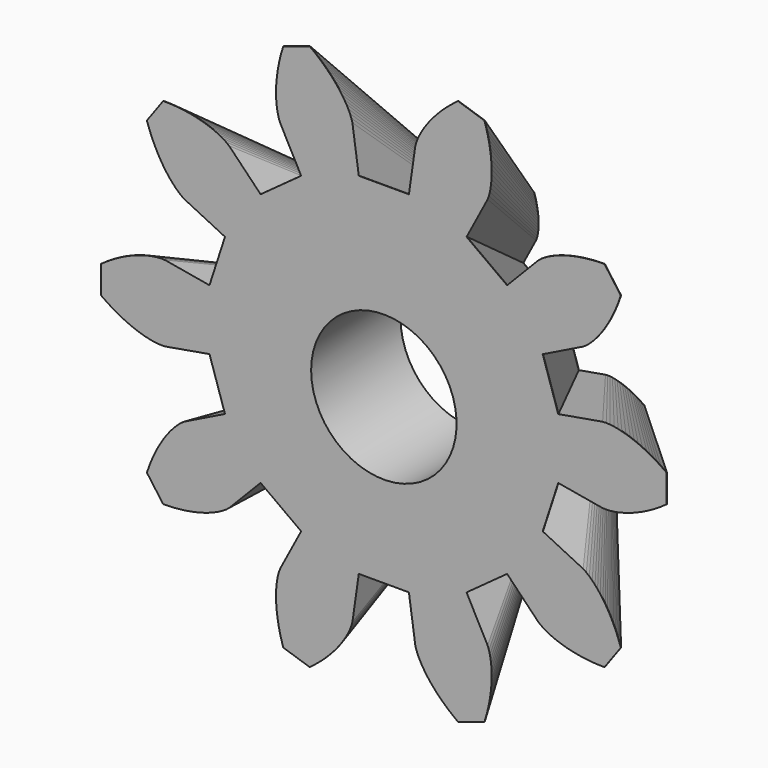
from build123d import *

# Parameters (mm, degrees)
F1_DEPTH = 0.01
F3_SCALE = 0.6058
F5_R     = 1.9570867443
F6_DEPTH = 3.011


# Not quite as in the source:
# - ends of sketch curves that miss each other by under 0.0002 mm in the source are joined


with BuildPart() as f1:
    # F0 (on Front) → F1 (new body)
    with BuildSketch(Plane.XZ):
        with BuildLine():
            ThreePointArc((4.2753417889, -0.9237346066), (4.4837280553, -0.2822940953), (4.6921702972, 0.3591282284))
            Line((4.6921702972, 0.3591282284), (5.878934, 0.152889))
            Line((5.878934, 0.152889), (5.978914, 0.147897))
            Line((5.978914, 0.147897), (6.083031, 0.153397))
            Line((6.083031, 0.153397), (6.188792, 0.166293))
            Line((6.188792, 0.166293), (6.296123, 0.185564))
            Line((6.296123, 0.185564), (6.39688, 0.208667))
            Line((6.39688, 0.208667), (6.507485, 0.239158))
            Line((6.507485, 0.239158), (6.627466, 0.277934))
            Line((6.627466, 0.277934), (6.729844, 0.315505))
            Line((6.729844, 0.315505), (6.837582, 0.359366))
            Line((6.837582, 0.359366), (6.95036, 0.409935))
            Line((6.95036, 0.409935), (7.067828, 0.467611))
            Line((7.067828, 0.467611), (7.158791, 0.515766))
            Line((7.158791, 0.515766), (7.252025, 0.568292))
            Line((7.252025, 0.568292), (7.347362, 0.62534))
            Line((7.347362, 0.62534), (7.444626, 0.687056))
            Line((7.444626, 0.687056), (7.610854, 0.801339))
            Line((7.610854, 0.801339), (7.610854, 1.547781))
            Line((7.610854, 1.547781), (7.444624, 1.662064))
            Line((7.444624, 1.662064), (7.347361, 1.723779))
            Line((7.347361, 1.723779), (7.252025, 1.780827))
            Line((7.252025, 1.780827), (7.15879, 1.833354))
            Line((7.15879, 1.833354), (7.067828, 1.881508))
            Line((7.067828, 1.881508), (6.950358, 1.939185))
            Line((6.950358, 1.939185), (6.837582, 1.989753))
            Line((6.837582, 1.989753), (6.729843, 2.033614))
            Line((6.729843, 2.033614), (6.627464, 2.071186))
            Line((6.627464, 2.071186), (6.507485, 2.109962))
            Line((6.507485, 2.109962), (6.39688, 2.140452))
            Line((6.39688, 2.140452), (6.296123, 2.163555))
            Line((6.296123, 2.163555), (6.188792, 2.182826))
            Line((6.188792, 2.182826), (6.08303, 2.195722))
            Line((6.08303, 2.195722), (5.978914, 2.201222))
            Line((5.978914, 2.201222), (5.878933, 2.19623))
            Line((5.878933, 2.19623), (4.692172, 1.989989))
            ThreePointArc((4.692172, 1.989989), (4.4837309325, 2.6314120428), (4.2753451638, 3.2728530532))
            Line((4.2753451638, 3.2728530532), (5.35668, 3.80356))
            Line((5.35668, 3.80356), (5.4405, 3.858289))
            Line((5.4405, 3.858289), (5.5215, 3.923937))
            Line((5.5215, 3.923937), (5.599482, 3.996535))
            Line((5.599482, 3.996535), (5.674988, 4.075213))
            Line((5.674988, 4.075213), (5.742922, 4.153126))
            Line((5.742922, 4.153126), (5.814482, 4.242806))
            Line((5.814482, 4.242806), (5.888756, 4.344699))
            Line((5.888756, 4.344699), (5.949498, 4.435272))
            Line((5.949498, 4.435272), (6.010879, 4.534083))
            Line((6.010879, 4.534083), (6.072394, 4.641282))
            Line((6.072394, 4.641282), (6.133527, 4.75699))
            Line((6.133527, 4.75699), (6.178813, 4.849415))
            Line((6.178813, 4.849415), (6.223367, 4.946711))
            Line((6.223367, 4.946711), (6.266963, 5.048901))
            Line((6.266963, 5.048901), (6.309377, 5.156001))
            Line((6.309377, 5.156001), (6.376684, 5.346164))
            Line((6.376684, 5.346164), (5.937936, 5.950048))
            Line((5.937936, 5.950048), (5.73628, 5.944798))
            Line((5.73628, 5.944798), (5.621317, 5.937556))
            Line((5.621317, 5.937556), (5.510656, 5.927672))
            Line((5.510656, 5.927672), (5.404354, 5.915365))
            Line((5.404354, 5.915365), (5.302459, 5.900857))
            Line((5.302459, 5.900857), (5.173523, 5.878471))
            Line((5.173523, 5.878471), (5.052562, 5.853093))
            Line((5.052562, 5.853093), (4.939618, 5.825251))
            Line((4.939618, 5.825251), (4.834708, 5.79547))
            Line((4.834708, 5.79547), (4.714851, 5.756318))
            Line((4.714851, 5.756318), (4.607447, 5.715973))
            Line((4.607447, 5.715973), (4.512354, 5.67544))
            Line((4.512354, 5.67544), (4.414194, 5.627943))
            Line((4.414194, 5.627943), (4.321051, 5.576212))
            Line((4.321051, 5.576212), (4.233586, 5.519463))
            Line((4.233586, 5.519463), (4.155634, 5.456658))
            Line((4.155634, 5.456658), (3.31675, 4.592245))
            ThreePointArc((3.31675, 4.592245), (2.7710979645, 4.9886473644), (2.2254808469, 5.3850977893))
            Line((2.2254808469, 5.3850977893), (2.788358, 6.450042))
            Line((2.788358, 6.450042), (2.824001, 6.543587))
            Line((2.824001, 6.543587), (2.850944, 6.644307))
            Line((2.850944, 6.644307), (2.871361, 6.748877))
            Line((2.871361, 6.748877), (2.886201, 6.856911))
            Line((2.886201, 6.856911), (2.895364, 6.959874))
            Line((2.895364, 6.959874), (2.900545, 7.074489))
            Line((2.900545, 7.074489), (2.900742, 7.200579))
            Line((2.900742, 7.200579), (2.896647, 7.309556))
            Line((2.896647, 7.309556), (2.888225, 7.425575))
            Line((2.888225, 7.425575), (2.874982, 7.548459))
            Line((2.874982, 7.548459), (2.856428, 7.678002))
            Line((2.856428, 7.678002), (2.83874, 7.779394))
            Line((2.83874, 7.779394), (2.817595, 7.884296))
            Line((2.817595, 7.884296), (2.792799, 7.992596))
            Line((2.792799, 7.992596), (2.76416, 8.10417))
            Line((2.76416, 8.10417), (2.706839, 8.297578))
            Line((2.706839, 8.297578), (1.99693, 8.528241))
            Line((1.99693, 8.528241), (1.836873, 8.405463))
            Line((1.836873, 8.405463), (1.748122, 8.332031))
            Line((1.748122, 8.332031), (1.664405, 8.258989))
            Line((1.664405, 8.258989), (1.585639, 8.186549))
            Line((1.585639, 8.186549), (1.511732, 8.11492))
            Line((1.511732, 8.11492), (1.420578, 8.021022))
            Line((1.420578, 8.021022), (1.337635, 7.929392))
            Line((1.337635, 7.929392), (1.262627, 7.840481))
            Line((1.262627, 7.840481), (1.195258, 7.754723))
            Line((1.195258, 7.754723), (1.121305, 7.652599))
            Line((1.121305, 7.652599), (1.058128, 7.556829))
            Line((1.058128, 7.556829), (1.00502, 7.468143))
            Line((1.00502, 7.468143), (0.953525, 7.37202))
            Line((0.953525, 7.37202), (0.908577, 7.27542))
            Line((0.908577, 7.27542), (0.871173, 7.178099))
            Line((0.871173, 7.178099), (0.845025, 7.081469))
            Line((0.845025, 7.081469), (0.674443, 5.88906))
            ThreePointArc((0.674443, 5.88906), (1.5e-06, 5.8890320012), (-0.67444, 5.8890618078))
            Line((-0.67444, 5.8890618078), (-0.845022, 7.08147))
            Line((-0.845022, 7.08147), (-0.87117, 7.178099))
            Line((-0.87117, 7.178099), (-0.908574, 7.27542))
            Line((-0.908574, 7.27542), (-0.953521, 7.37202))
            Line((-0.953521, 7.37202), (-1.005016, 7.468143))
            Line((-1.005016, 7.468143), (-1.058124, 7.556829))
            Line((-1.058124, 7.556829), (-1.121301, 7.652598))
            Line((-1.121301, 7.652598), (-1.195255, 7.754725))
            Line((-1.195255, 7.754725), (-1.262624, 7.840481))
            Line((-1.262624, 7.840481), (-1.337632, 7.929392))
            Line((-1.337632, 7.929392), (-1.420575, 8.021024))
            Line((-1.420575, 8.021024), (-1.511728, 8.11492))
            Line((-1.511728, 8.11492), (-1.585636, 8.186551))
            Line((-1.585636, 8.186551), (-1.664402, 8.25899))
            Line((-1.664402, 8.25899), (-1.748119, 8.332032))
            Line((-1.748119, 8.332032), (-1.83687, 8.405464))
            Line((-1.83687, 8.405464), (-1.996926, 8.528241))
            Line((-1.996926, 8.528241), (-2.706835, 8.297578))
            Line((-2.706835, 8.297578), (-2.764157, 8.104169))
            Line((-2.764157, 8.104169), (-2.792795, 7.992595))
            Line((-2.792795, 7.992595), (-2.817591, 7.884296))
            Line((-2.817591, 7.884296), (-2.838736, 7.779392))
            Line((-2.838736, 7.779392), (-2.856425, 7.678002))
            Line((-2.856425, 7.678002), (-2.874978, 7.548459))
            Line((-2.874978, 7.548459), (-2.888221, 7.425576))
            Line((-2.888221, 7.425576), (-2.896643, 7.309556))
            Line((-2.896643, 7.309556), (-2.900739, 7.200578))
            Line((-2.900739, 7.200578), (-2.900542, 7.074489))
            Line((-2.900542, 7.074489), (-2.895361, 6.959875))
            Line((-2.895361, 6.959875), (-2.886197, 6.856911))
            Line((-2.886197, 6.856911), (-2.871358, 6.748877))
            Line((-2.871358, 6.748877), (-2.850941, 6.644307))
            Line((-2.850941, 6.644307), (-2.823998, 6.543587))
            Line((-2.823998, 6.543587), (-2.788355, 6.450042))
            Line((-2.788355, 6.450042), (-2.225478, 5.385097))
            ThreePointArc((-2.225478, 5.385097), (-2.771095971, 4.9886482498), (-3.3167477562, 4.592246041))
            Line((-3.3167477562, 4.592246041), (-4.155632, 5.456658))
            Line((-4.155632, 5.456658), (-4.233584, 5.519464))
            Line((-4.233584, 5.519464), (-4.321049, 5.576213))
            Line((-4.321049, 5.576213), (-4.414192, 5.627944))
            Line((-4.414192, 5.627944), (-4.512352, 5.675442))
            Line((-4.512352, 5.675442), (-4.607445, 5.715974))
            Line((-4.607445, 5.715974), (-4.714848, 5.756319))
            Line((-4.714848, 5.756319), (-4.834706, 5.795471))
            Line((-4.834706, 5.795471), (-4.939616, 5.825252))
            Line((-4.939616, 5.825252), (-5.052559, 5.853094))
            Line((-5.052559, 5.853094), (-5.173522, 5.878472))
            Line((-5.173522, 5.878472), (-5.302457, 5.900857))
            Line((-5.302457, 5.900857), (-5.404352, 5.915366))
            Line((-5.404352, 5.915366), (-5.510654, 5.927673))
            Line((-5.510654, 5.927673), (-5.621316, 5.937558))
            Line((-5.621316, 5.937558), (-5.736279, 5.944799))
            Line((-5.736279, 5.944799), (-5.937934, 5.950049))
            Line((-5.937934, 5.950049), (-6.376683, 5.346165))
            Line((-6.376683, 5.346165), (-6.309373, 5.156001))
            Line((-6.309373, 5.156001), (-6.266961, 5.048902))
            Line((-6.266961, 5.048902), (-6.223364, 4.946712))
            Line((-6.223364, 4.946712), (-6.17881, 4.849415))
            Line((-6.17881, 4.849415), (-6.133525, 4.756991))
            Line((-6.133525, 4.756991), (-6.072391, 4.641283))
            Line((-6.072391, 4.641283), (-6.010877, 4.534084))
            Line((-6.010877, 4.534084), (-5.949495, 4.435272))
            Line((-5.949495, 4.435272), (-5.888753, 4.344699))
            Line((-5.888753, 4.344699), (-5.81448, 4.242807))
            Line((-5.81448, 4.242807), (-5.74292, 4.153128))
            Line((-5.74292, 4.153128), (-5.674986, 4.075214))
            Line((-5.674986, 4.075214), (-5.59948, 3.996536))
            Line((-5.59948, 3.996536), (-5.521498, 3.923937))
            Line((-5.521498, 3.923937), (-5.440498, 3.85829))
            Line((-5.440498, 3.85829), (-5.356678, 3.803561))
            Line((-5.356678, 3.803561), (-4.275343, 3.272853))
            ThreePointArc((-4.275343, 3.272853), (-4.4837282639, 2.6314121631), (-4.6921703347, 1.9899897838))
            Line((-4.6921703347, 1.9899897838), (-5.878932, 2.196231))
            Line((-5.878932, 2.196231), (-5.978913, 2.201222))
            Line((-5.978913, 2.201222), (-6.08303, 2.195723))
            Line((-6.08303, 2.195723), (-6.188791, 2.182826))
            Line((-6.188791, 2.182826), (-6.296122, 2.163555))
            Line((-6.296122, 2.163555), (-6.396879, 2.140453))
            Line((-6.396879, 2.140453), (-6.507485, 2.109962))
            Line((-6.507485, 2.109962), (-6.627465, 2.071186))
            Line((-6.627465, 2.071186), (-6.729843, 2.033615))
            Line((-6.729843, 2.033615), (-6.837581, 1.989753))
            Line((-6.837581, 1.989753), (-6.950359, 1.939185))
            Line((-6.950359, 1.939185), (-7.067828, 1.881509))
            Line((-7.067828, 1.881509), (-7.158791, 1.833354))
            Line((-7.158791, 1.833354), (-7.252025, 1.780828))
            Line((-7.252025, 1.780828), (-7.347361, 1.723779))
            Line((-7.347361, 1.723779), (-7.444625, 1.662064))
            Line((-7.444625, 1.662064), (-7.610853, 1.547781))
            Line((-7.610853, 1.547781), (-7.610853, 0.801339))
            Line((-7.610853, 0.801339), (-7.444624, 0.687056))
            Line((-7.444624, 0.687056), (-7.34736, 0.625341))
            Line((-7.34736, 0.625341), (-7.252024, 0.568293))
            Line((-7.252024, 0.568293), (-7.158789, 0.515766))
            Line((-7.158789, 0.515766), (-7.067828, 0.467612))
            Line((-7.067828, 0.467612), (-6.950358, 0.409935))
            Line((-6.950358, 0.409935), (-6.837581, 0.359367))
            Line((-6.837581, 0.359367), (-6.729843, 0.315506))
            Line((-6.729843, 0.315506), (-6.627464, 0.277934))
            Line((-6.627464, 0.277934), (-6.507485, 0.239159))
            Line((-6.507485, 0.239159), (-6.396879, 0.208668))
            Line((-6.396879, 0.208668), (-6.296122, 0.185565))
            Line((-6.296122, 0.185565), (-6.18879, 0.166294))
            Line((-6.18879, 0.166294), (-6.083029, 0.153398))
            Line((-6.083029, 0.153398), (-5.978913, 0.147898))
            Line((-5.978913, 0.147898), (-5.878932, 0.15289))
            Line((-5.878932, 0.15289), (-4.692171, 0.359131))
            ThreePointArc((-4.692171, 0.359131), (-4.4837298858, -0.2822915276), (-4.2753442362, -0.9237320767))
            Line((-4.2753442362, -0.9237320767), (-5.356681, -1.45444))
            Line((-5.356681, -1.45444), (-5.440501, -1.509168))
            Line((-5.440501, -1.509168), (-5.5215, -1.574816))
            Line((-5.5215, -1.574816), (-5.599482, -1.647414))
            Line((-5.599482, -1.647414), (-5.674988, -1.726092))
            Line((-5.674988, -1.726092), (-5.742923, -1.804005))
            Line((-5.742923, -1.804005), (-5.814482, -1.893685))
            Line((-5.814482, -1.893685), (-5.888757, -1.995578))
            Line((-5.888757, -1.995578), (-5.949499, -2.08615))
            Line((-5.949499, -2.08615), (-6.010879, -2.184962))
            Line((-6.010879, -2.184962), (-6.072395, -2.292162))
            Line((-6.072395, -2.292162), (-6.133528, -2.407869))
            Line((-6.133528, -2.407869), (-6.178814, -2.500294))
            Line((-6.178814, -2.500294), (-6.223368, -2.59759))
            Line((-6.223368, -2.59759), (-6.266964, -2.69978))
            Line((-6.266964, -2.69978), (-6.309378, -2.80688))
            Line((-6.309378, -2.80688), (-6.376685, -2.997043))
            Line((-6.376685, -2.997043), (-5.937937, -3.600927))
            Line((-5.937937, -3.600927), (-5.736281, -3.595677))
            Line((-5.736281, -3.595677), (-5.621318, -3.588435))
            Line((-5.621318, -3.588435), (-5.510657, -3.578551))
            Line((-5.510657, -3.578551), (-5.404354, -3.566244))
            Line((-5.404354, -3.566244), (-5.30246, -3.551736))
            Line((-5.30246, -3.551736), (-5.173523, -3.52935))
            Line((-5.173523, -3.52935), (-5.052562, -3.503972))
            Line((-5.052562, -3.503972), (-4.939619, -3.47613))
            Line((-4.939619, -3.47613), (-4.834708, -3.446349))
            Line((-4.834708, -3.446349), (-4.714851, -3.407198))
            Line((-4.714851, -3.407198), (-4.607448, -3.366853))
            Line((-4.607448, -3.366853), (-4.512355, -3.32632))
            Line((-4.512355, -3.32632), (-4.414194, -3.278822))
            Line((-4.414194, -3.278822), (-4.321052, -3.227091))
            Line((-4.321052, -3.227091), (-4.233587, -3.170342))
            Line((-4.233587, -3.170342), (-4.155635, -3.107537))
            Line((-4.155635, -3.107537), (-3.31675, -2.243124))
            ThreePointArc((-3.31675, -2.243124), (-2.7710983472, -2.6395268912), (-2.2254812543, -3.0359773499))
            Line((-2.2254812543, -3.0359773499), (-2.788359, -4.100922))
            Line((-2.788359, -4.100922), (-2.824002, -4.194467))
            Line((-2.824002, -4.194467), (-2.850945, -4.295187))
            Line((-2.850945, -4.295187), (-2.871362, -4.399757))
            Line((-2.871362, -4.399757), (-2.886201, -4.50779))
            Line((-2.886201, -4.50779), (-2.895365, -4.610754))
            Line((-2.895365, -4.610754), (-2.900546, -4.725369))
            Line((-2.900546, -4.725369), (-2.900744, -4.851459))
            Line((-2.900744, -4.851459), (-2.896648, -4.960437))
            Line((-2.896648, -4.960437), (-2.888226, -5.076456))
            Line((-2.888226, -5.076456), (-2.874983, -5.19934))
            Line((-2.874983, -5.19934), (-2.856429, -5.328883))
            Line((-2.856429, -5.328883), (-2.838741, -5.430275))
            Line((-2.838741, -5.430275), (-2.817596, -5.535177))
            Line((-2.817596, -5.535177), (-2.7928, -5.643476))
            Line((-2.7928, -5.643476), (-2.764162, -5.75505))
            Line((-2.764162, -5.75505), (-2.70684, -5.948458))
            Line((-2.70684, -5.948458), (-1.996931, -6.179121))
            Line((-1.996931, -6.179121), (-1.836874, -6.056343))
            Line((-1.836874, -6.056343), (-1.748123, -5.982912))
            Line((-1.748123, -5.982912), (-1.664406, -5.90987))
            Line((-1.664406, -5.90987), (-1.585639, -5.83743))
            Line((-1.585639, -5.83743), (-1.511733, -5.765801))
            Line((-1.511733, -5.765801), (-1.420579, -5.671903))
            Line((-1.420579, -5.671903), (-1.337636, -5.580273))
            Line((-1.337636, -5.580273), (-1.262628, -5.491361))
            Line((-1.262628, -5.491361), (-1.195259, -5.405603))
            Line((-1.195259, -5.405603), (-1.121305, -5.303479))
            Line((-1.121305, -5.303479), (-1.058128, -5.207709))
            Line((-1.058128, -5.207709), (-1.00502, -5.119023))
            Line((-1.00502, -5.119023), (-0.953526, -5.0229))
            Line((-0.953526, -5.0229), (-0.908578, -4.9263))
            Line((-0.908578, -4.9263), (-0.871174, -4.828979))
            Line((-0.871174, -4.828979), (-0.845026, -4.73235))
            Line((-0.845026, -4.73235), (-0.674443, -3.539941))
            ThreePointArc((-0.674443, -3.539941), (-1.5e-06, -3.5399120003), (0.67444, -3.5399416176))
            Line((0.67444, -3.5399416176), (0.845021, -4.732351))
            Line((0.845021, -4.732351), (0.87117, -4.82898))
            Line((0.87117, -4.82898), (0.908574, -4.926302))
            Line((0.908574, -4.926302), (0.953521, -5.022901))
            Line((0.953521, -5.022901), (1.005016, -5.119024))
            Line((1.005016, -5.119024), (1.058123, -5.20771))
            Line((1.058123, -5.20771), (1.1213, -5.30348))
            Line((1.1213, -5.30348), (1.195254, -5.405606))
            Line((1.195254, -5.405606), (1.262623, -5.491364))
            Line((1.262623, -5.491364), (1.337631, -5.580275))
            Line((1.337631, -5.580275), (1.420574, -5.671906))
            Line((1.420574, -5.671906), (1.511728, -5.765803))
            Line((1.511728, -5.765803), (1.585635, -5.837433))
            Line((1.585635, -5.837433), (1.664401, -5.909872))
            Line((1.664401, -5.909872), (1.748118, -5.982913))
            Line((1.748118, -5.982913), (1.836869, -6.056346))
            Line((1.836869, -6.056346), (1.996925, -6.179123))
            Line((1.996925, -6.179123), (2.706834, -5.94846))
            Line((2.706834, -5.94846), (2.764156, -5.755051))
            Line((2.764156, -5.755051), (2.792795, -5.643476))
            Line((2.792795, -5.643476), (2.817591, -5.535178))
            Line((2.817591, -5.535178), (2.838735, -5.430275))
            Line((2.838735, -5.430275), (2.856424, -5.328885))
            Line((2.856424, -5.328885), (2.874977, -5.199341))
            Line((2.874977, -5.199341), (2.888221, -5.076458))
            Line((2.888221, -5.076458), (2.896643, -4.960438))
            Line((2.896643, -4.960438), (2.900738, -4.851459))
            Line((2.900738, -4.851459), (2.900541, -4.725371))
            Line((2.900541, -4.725371), (2.89536, -4.610756))
            Line((2.89536, -4.610756), (2.886197, -4.507792))
            Line((2.886197, -4.507792), (2.871357, -4.399759))
            Line((2.871357, -4.399759), (2.850941, -4.295188))
            Line((2.850941, -4.295188), (2.823998, -4.194468))
            Line((2.823998, -4.194468), (2.788354, -4.100924))
            Line((2.788354, -4.100924), (2.225479, -3.035979))
            ThreePointArc((2.225479, -3.035979), (2.7710963565, -2.6395289039), (3.3167481995, -2.2431262746))
            Line((3.3167481995, -2.2431262746), (4.155631, -3.10754))
            Line((4.155631, -3.10754), (4.233583, -3.170346))
            Line((4.233583, -3.170346), (4.321048, -3.227095))
            Line((4.321048, -3.227095), (4.41419, -3.278826))
            Line((4.41419, -3.278826), (4.51235, -3.326324))
            Line((4.51235, -3.326324), (4.607444, -3.366856))
            Line((4.607444, -3.366856), (4.714847, -3.407201))
            Line((4.714847, -3.407201), (4.834705, -3.446354))
            Line((4.834705, -3.446354), (4.939615, -3.476134))
            Line((4.939615, -3.476134), (5.052558, -3.503976))
            Line((5.052558, -3.503976), (5.17352, -3.529355))
            Line((5.17352, -3.529355), (5.302456, -3.55174))
            Line((5.302456, -3.55174), (5.404351, -3.566249))
            Line((5.404351, -3.566249), (5.510653, -3.578556))
            Line((5.510653, -3.578556), (5.621314, -3.58844))
            Line((5.621314, -3.58844), (5.736278, -3.595682))
            Line((5.736278, -3.595682), (5.937933, -3.600932))
            Line((5.937933, -3.600932), (6.376681, -2.997048))
            Line((6.376681, -2.997048), (6.309372, -2.806883))
            Line((6.309372, -2.806883), (6.26696, -2.699785))
            Line((6.26696, -2.699785), (6.223363, -2.597595))
            Line((6.223363, -2.597595), (6.178809, -2.500297))
            Line((6.178809, -2.500297), (6.133524, -2.407874))
            Line((6.133524, -2.407874), (6.07239, -2.292165))
            Line((6.07239, -2.292165), (6.010875, -2.184966))
            Line((6.010875, -2.184966), (5.949495, -2.086155))
            Line((5.949495, -2.086155), (5.888752, -1.995582))
            Line((5.888752, -1.995582), (5.814479, -1.89369))
            Line((5.814479, -1.89369), (5.742919, -1.80401))
            Line((5.742919, -1.80401), (5.674985, -1.726096))
            Line((5.674985, -1.726096), (5.599479, -1.647418))
            Line((5.599479, -1.647418), (5.521497, -1.574819))
            Line((5.521497, -1.574819), (5.440498, -1.509172))
            Line((5.440498, -1.509172), (5.356677, -1.454443))
            Line((5.356677, -1.454443), (4.2753417889, -0.9237346066))
        make_face()
    extrude(amount=F1_DEPTH)


with BuildPart() as f2_1:
    # F2: copy of F1
    add(f1.part.moved(Location((0, -3, 0))))


with BuildPart() as f1_1:
    # F3: moved
    add(f1.part.scale(F3_SCALE))


with BuildPart() as f4:
    # F2_face (on face) → F4 section 0
    with BuildSketch(Plane(origin=(1.724e-07, -3, 1.1745596089), x_dir=(-1, 0, 0), z_dir=(0, 1, 0))):
        with BuildLine():
            ThreePointArc((-4.6921701248, -0.8154313805), (-4.4837278829, -1.4568537042), (-4.2753416165, -2.0982942155))
            Line((-4.2753416165, -2.0982942155), (-5.3566768276, -2.6290026089))
            Line((-5.3566768276, -2.6290026089), (-5.4404978276, -2.6837316089))
            Line((-5.4404978276, -2.6837316089), (-5.5214968276, -2.7493786089))
            Line((-5.5214968276, -2.7493786089), (-5.5994788276, -2.8219776089))
            Line((-5.5994788276, -2.8219776089), (-5.6749848276, -2.9006556089))
            Line((-5.6749848276, -2.9006556089), (-5.7429188276, -2.9785696089))
            Line((-5.7429188276, -2.9785696089), (-5.8144788276, -3.0682496089))
            Line((-5.8144788276, -3.0682496089), (-5.8887518276, -3.1701416089))
            Line((-5.8887518276, -3.1701416089), (-5.9494948276, -3.2607146089))
            Line((-5.9494948276, -3.2607146089), (-6.0108748276, -3.3595256089))
            Line((-6.0108748276, -3.3595256089), (-6.0723898276, -3.4667246089))
            Line((-6.0723898276, -3.4667246089), (-6.1335238276, -3.5824336089))
            Line((-6.1335238276, -3.5824336089), (-6.1788088276, -3.6748566089))
            Line((-6.1788088276, -3.6748566089), (-6.2233628276, -3.7721546089))
            Line((-6.2233628276, -3.7721546089), (-6.2669598276, -3.8743446089))
            Line((-6.2669598276, -3.8743446089), (-6.3093718276, -3.9814426089))
            Line((-6.3093718276, -3.9814426089), (-6.3766808276, -4.1716076089))
            Line((-6.3766808276, -4.1716076089), (-5.9379328276, -4.7754916089))
            Line((-5.9379328276, -4.7754916089), (-5.7362778276, -4.7702416089))
            Line((-5.7362778276, -4.7702416089), (-5.6213138276, -4.7629996089))
            Line((-5.6213138276, -4.7629996089), (-5.5106528276, -4.7531156089))
            Line((-5.5106528276, -4.7531156089), (-5.4043508276, -4.7408086089))
            Line((-5.4043508276, -4.7408086089), (-5.3024558276, -4.7262996089))
            Line((-5.3024558276, -4.7262996089), (-5.1735198276, -4.7039146089))
            Line((-5.1735198276, -4.7039146089), (-5.0525578276, -4.6785356089))
            Line((-5.0525578276, -4.6785356089), (-4.9396148276, -4.6506936089))
            Line((-4.9396148276, -4.6506936089), (-4.8347048276, -4.6209136089))
            Line((-4.8347048276, -4.6209136089), (-4.7148468276, -4.5817606089))
            Line((-4.7148468276, -4.5817606089), (-4.6074438276, -4.5414156089))
            Line((-4.6074438276, -4.5414156089), (-4.5123498276, -4.5008836089))
            Line((-4.5123498276, -4.5008836089), (-4.4141898276, -4.4533856089))
            Line((-4.4141898276, -4.4533856089), (-4.3210478276, -4.4016546089))
            Line((-4.3210478276, -4.4016546089), (-4.2335828276, -4.3449056089))
            Line((-4.2335828276, -4.3449056089), (-4.1556308276, -4.2820996089))
            Line((-4.1556308276, -4.2820996089), (-3.3167480271, -3.4176858835))
            ThreePointArc((-3.3167480271, -3.4176858835), (-2.7710961841, -3.8140885128), (-2.2254788276, -4.2105386089))
            Line((-2.2254788276, -4.2105386089), (-2.7883538276, -5.2754836089))
            Line((-2.7883538276, -5.2754836089), (-2.8239978276, -5.3690276089))
            Line((-2.8239978276, -5.3690276089), (-2.8509408276, -5.4697476089))
            Line((-2.8509408276, -5.4697476089), (-2.8713568276, -5.5743186089))
            Line((-2.8713568276, -5.5743186089), (-2.8861968276, -5.6823516089))
            Line((-2.8861968276, -5.6823516089), (-2.8953598276, -5.7853156089))
            Line((-2.8953598276, -5.7853156089), (-2.9005408276, -5.8999306089))
            Line((-2.9005408276, -5.8999306089), (-2.9007378276, -6.0260186089))
            Line((-2.9007378276, -6.0260186089), (-2.8966428276, -6.1349976089))
            Line((-2.8966428276, -6.1349976089), (-2.8882208276, -6.2510176089))
            Line((-2.8882208276, -6.2510176089), (-2.8749768276, -6.3739006089))
            Line((-2.8749768276, -6.3739006089), (-2.8564238276, -6.5034446089))
            Line((-2.8564238276, -6.5034446089), (-2.8387348276, -6.6048346089))
            Line((-2.8387348276, -6.6048346089), (-2.8175908276, -6.7097376089))
            Line((-2.8175908276, -6.7097376089), (-2.7927948276, -6.8180356089))
            Line((-2.7927948276, -6.8180356089), (-2.7641558276, -6.9296106089))
            Line((-2.7641558276, -6.9296106089), (-2.7068338276, -7.1230196089))
            Line((-2.7068338276, -7.1230196089), (-1.9969248276, -7.3536826089))
            Line((-1.9969248276, -7.3536826089), (-1.8368688276, -7.2309056089))
            Line((-1.8368688276, -7.2309056089), (-1.7481178276, -7.1574726089))
            Line((-1.7481178276, -7.1574726089), (-1.6644008276, -7.0844316089))
            Line((-1.6644008276, -7.0844316089), (-1.5856348276, -7.0119926089))
            Line((-1.5856348276, -7.0119926089), (-1.5117278276, -6.9403626089))
            Line((-1.5117278276, -6.9403626089), (-1.4205738276, -6.8464656089))
            Line((-1.4205738276, -6.8464656089), (-1.3376308276, -6.7548346089))
            Line((-1.3376308276, -6.7548346089), (-1.2626228276, -6.6659236089))
            Line((-1.2626228276, -6.6659236089), (-1.1952538276, -6.5801656089))
            Line((-1.1952538276, -6.5801656089), (-1.1212998276, -6.4780396089))
            Line((-1.1212998276, -6.4780396089), (-1.0581228276, -6.3822696089))
            Line((-1.0581228276, -6.3822696089), (-1.0050158276, -6.2935836089))
            Line((-1.0050158276, -6.2935836089), (-0.9535208276, -6.1974606089))
            Line((-0.9535208276, -6.1974606089), (-0.9085738276, -6.1008616089))
            Line((-0.9085738276, -6.1008616089), (-0.8711698276, -6.0035396089))
            Line((-0.8711698276, -6.0035396089), (-0.8450208276, -5.9069106089))
            Line((-0.8450208276, -5.9069106089), (-0.6744398276, -4.7145012265))
            ThreePointArc((-0.6744398276, -4.7145012265), (1.6724e-06, -4.7144716092), (0.6744431724, -4.7145006089))
            Line((0.6744431724, -4.7145006089), (0.8450261724, -5.9069096089))
            Line((0.8450261724, -5.9069096089), (0.8711741724, -6.0035386089))
            Line((0.8711741724, -6.0035386089), (0.9085781724, -6.1008596089))
            Line((0.9085781724, -6.1008596089), (0.9535261724, -6.1974596089))
            Line((0.9535261724, -6.1974596089), (1.0050201724, -6.2935826089))
            Line((1.0050201724, -6.2935826089), (1.0581281724, -6.3822686089))
            Line((1.0581281724, -6.3822686089), (1.1213051724, -6.4780386089))
            Line((1.1213051724, -6.4780386089), (1.1952591724, -6.5801626089))
            Line((1.1952591724, -6.5801626089), (1.2626281724, -6.6659206089))
            Line((1.2626281724, -6.6659206089), (1.3376361724, -6.7548326089))
            Line((1.3376361724, -6.7548326089), (1.4205791724, -6.8464626089))
            Line((1.4205791724, -6.8464626089), (1.5117331724, -6.9403606089))
            Line((1.5117331724, -6.9403606089), (1.5856391724, -7.0119896089))
            Line((1.5856391724, -7.0119896089), (1.6644061724, -7.0844296089))
            Line((1.6644061724, -7.0844296089), (1.7481231724, -7.1574716089))
            Line((1.7481231724, -7.1574716089), (1.8368741724, -7.2309026089))
            Line((1.8368741724, -7.2309026089), (1.9969311724, -7.3536806089))
            Line((1.9969311724, -7.3536806089), (2.7068401724, -7.1230176089))
            Line((2.7068401724, -7.1230176089), (2.7641621724, -6.9296096089))
            Line((2.7641621724, -6.9296096089), (2.7928001724, -6.8180356089))
            Line((2.7928001724, -6.8180356089), (2.8175961724, -6.7097366089))
            Line((2.8175961724, -6.7097366089), (2.8387411724, -6.6048346089))
            Line((2.8387411724, -6.6048346089), (2.8564291724, -6.5034426089))
            Line((2.8564291724, -6.5034426089), (2.8749831724, -6.3738996089))
            Line((2.8749831724, -6.3738996089), (2.8882261724, -6.2510156089))
            Line((2.8882261724, -6.2510156089), (2.8966481724, -6.1349966089))
            Line((2.8966481724, -6.1349966089), (2.9007441724, -6.0260186089))
            Line((2.9007441724, -6.0260186089), (2.9005461724, -5.8999286089))
            Line((2.9005461724, -5.8999286089), (2.8953651724, -5.7853136089))
            Line((2.8953651724, -5.7853136089), (2.8862011724, -5.6823496089))
            Line((2.8862011724, -5.6823496089), (2.8713621724, -5.5743166089))
            Line((2.8713621724, -5.5743166089), (2.8509451724, -5.4697466089))
            Line((2.8509451724, -5.4697466089), (2.8240021724, -5.3690266089))
            Line((2.8240021724, -5.3690266089), (2.7883591724, -5.2754816089))
            Line((2.7883591724, -5.2754816089), (2.2254814266, -4.2105369588))
            ThreePointArc((2.2254814266, -4.2105369588), (2.7710985196, -3.8140865), (3.3167501724, -3.4176836089))
            Line((3.3167501724, -3.4176836089), (4.1556351724, -4.2820966089))
            Line((4.1556351724, -4.2820966089), (4.2335871724, -4.3449016089))
            Line((4.2335871724, -4.3449016089), (4.3210521724, -4.4016506089))
            Line((4.3210521724, -4.4016506089), (4.4141941724, -4.4533816089))
            Line((4.4141941724, -4.4533816089), (4.5123551724, -4.5008796089))
            Line((4.5123551724, -4.5008796089), (4.6074481724, -4.5414126089))
            Line((4.6074481724, -4.5414126089), (4.7148511724, -4.5817576089))
            Line((4.7148511724, -4.5817576089), (4.8347081724, -4.6209086089))
            Line((4.8347081724, -4.6209086089), (4.9396191724, -4.6506896089))
            Line((4.9396191724, -4.6506896089), (5.0525621724, -4.6785316089))
            Line((5.0525621724, -4.6785316089), (5.1735231724, -4.7039096089))
            Line((5.1735231724, -4.7039096089), (5.3024601724, -4.7262956089))
            Line((5.3024601724, -4.7262956089), (5.4043541724, -4.7408036089))
            Line((5.4043541724, -4.7408036089), (5.5106571724, -4.7531106089))
            Line((5.5106571724, -4.7531106089), (5.6213181724, -4.7629946089))
            Line((5.6213181724, -4.7629946089), (5.7362811724, -4.7702366089))
            Line((5.7362811724, -4.7702366089), (5.9379371724, -4.7754866089))
            Line((5.9379371724, -4.7754866089), (6.3766851724, -4.1716026089))
            Line((6.3766851724, -4.1716026089), (6.3093781724, -3.9814396089))
            Line((6.3093781724, -3.9814396089), (6.2669641724, -3.8743396089))
            Line((6.2669641724, -3.8743396089), (6.2233681724, -3.7721496089))
            Line((6.2233681724, -3.7721496089), (6.1788141724, -3.6748536089))
            Line((6.1788141724, -3.6748536089), (6.1335281724, -3.5824286089))
            Line((6.1335281724, -3.5824286089), (6.0723951724, -3.4667216089))
            Line((6.0723951724, -3.4667216089), (6.0108791724, -3.3595216089))
            Line((6.0108791724, -3.3595216089), (5.9494991724, -3.2607096089))
            Line((5.9494991724, -3.2607096089), (5.8887571724, -3.1701376089))
            Line((5.8887571724, -3.1701376089), (5.8144821724, -3.0682446089))
            Line((5.8144821724, -3.0682446089), (5.7429231724, -2.9785646089))
            Line((5.7429231724, -2.9785646089), (5.6749881724, -2.9006516089))
            Line((5.6749881724, -2.9006516089), (5.5994821724, -2.8219736089))
            Line((5.5994821724, -2.8219736089), (5.5215001724, -2.7493756089))
            Line((5.5215001724, -2.7493756089), (5.4405011724, -2.6837276089))
            Line((5.4405011724, -2.6837276089), (5.3566811724, -2.6289996089))
            Line((5.3566811724, -2.6289996089), (4.2753444086, -2.0982916856))
            ThreePointArc((4.2753444086, -2.0982916856), (4.4837300582, -1.4568511365), (4.6921711724, -0.8154286089))
            Line((4.6921711724, -0.8154286089), (5.8789321724, -1.0216696089))
            Line((5.8789321724, -1.0216696089), (5.9789131724, -1.0266616089))
            Line((5.9789131724, -1.0266616089), (6.0830291724, -1.0211616089))
            Line((6.0830291724, -1.0211616089), (6.1887901724, -1.0082656089))
            Line((6.1887901724, -1.0082656089), (6.2961221724, -0.9889946089))
            Line((6.2961221724, -0.9889946089), (6.3968791724, -0.9658916089))
            Line((6.3968791724, -0.9658916089), (6.5074851724, -0.9354006089))
            Line((6.5074851724, -0.9354006089), (6.6274641724, -0.8966256089))
            Line((6.6274641724, -0.8966256089), (6.7298431724, -0.8590536089))
            Line((6.7298431724, -0.8590536089), (6.8375811724, -0.8151926089))
            Line((6.8375811724, -0.8151926089), (6.9503581724, -0.7646246089))
            Line((6.9503581724, -0.7646246089), (7.0678281724, -0.7069476089))
            Line((7.0678281724, -0.7069476089), (7.1587891724, -0.6587936089))
            Line((7.1587891724, -0.6587936089), (7.2520241724, -0.6062666089))
            Line((7.2520241724, -0.6062666089), (7.3473601724, -0.5492186089))
            Line((7.3473601724, -0.5492186089), (7.4446241724, -0.4875036089))
            Line((7.4446241724, -0.4875036089), (7.6108531724, -0.3732206089))
            Line((7.6108531724, -0.3732206089), (7.6108531724, 0.3732213911))
            Line((7.6108531724, 0.3732213911), (7.4446251724, 0.4875043911))
            Line((7.4446251724, 0.4875043911), (7.3473611724, 0.5492193911))
            Line((7.3473611724, 0.5492193911), (7.2520251724, 0.6062683911))
            Line((7.2520251724, 0.6062683911), (7.1587911724, 0.6587943911))
            Line((7.1587911724, 0.6587943911), (7.0678281724, 0.7069493911))
            Line((7.0678281724, 0.7069493911), (6.9503591724, 0.7646253911))
            Line((6.9503591724, 0.7646253911), (6.8375811724, 0.8151933911))
            Line((6.8375811724, 0.8151933911), (6.7298431724, 0.8590553911))
            Line((6.7298431724, 0.8590553911), (6.6274651724, 0.8966263911))
            Line((6.6274651724, 0.8966263911), (6.5074851724, 0.9354023911))
            Line((6.5074851724, 0.9354023911), (6.3968791724, 0.9658933911))
            Line((6.3968791724, 0.9658933911), (6.2961221724, 0.9889953911))
            Line((6.2961221724, 0.9889953911), (6.1887911724, 1.0082663911))
            Line((6.1887911724, 1.0082663911), (6.0830301724, 1.0211633911))
            Line((6.0830301724, 1.0211633911), (5.9789131724, 1.0266623911))
            Line((5.9789131724, 1.0266623911), (5.8789321724, 1.0216713911))
            Line((5.8789321724, 1.0216713911), (4.6921705071, 0.8154301749))
            ThreePointArc((4.6921705071, 0.8154301749), (4.4837284363, 1.4568525542), (4.2753431724, 2.0982933911))
            Line((4.2753431724, 2.0982933911), (5.3566781724, 2.6290013911))
            Line((5.3566781724, 2.6290013911), (5.4404981724, 2.6837303911))
            Line((5.4404981724, 2.6837303911), (5.5214981724, 2.7493773911))
            Line((5.5214981724, 2.7493773911), (5.5994801724, 2.8219763911))
            Line((5.5994801724, 2.8219763911), (5.6749861724, 2.9006543911))
            Line((5.6749861724, 2.9006543911), (5.7429201724, 2.9785683911))
            Line((5.7429201724, 2.9785683911), (5.8144801724, 3.0682473911))
            Line((5.8144801724, 3.0682473911), (5.8887531724, 3.1701393911))
            Line((5.8887531724, 3.1701393911), (5.9494951724, 3.2607123911))
            Line((5.9494951724, 3.2607123911), (6.0108771724, 3.3595243911))
            Line((6.0108771724, 3.3595243911), (6.0723911724, 3.4667233911))
            Line((6.0723911724, 3.4667233911), (6.1335251724, 3.5824313911))
            Line((6.1335251724, 3.5824313911), (6.1788101724, 3.6748553911))
            Line((6.1788101724, 3.6748553911), (6.2233641724, 3.7721523911))
            Line((6.2233641724, 3.7721523911), (6.2669611724, 3.8743423911))
            Line((6.2669611724, 3.8743423911), (6.3093731724, 3.9814413911))
            Line((6.3093731724, 3.9814413911), (6.3766831724, 4.1716053911))
            Line((6.3766831724, 4.1716053911), (5.9379341724, 4.7754893911))
            Line((5.9379341724, 4.7754893911), (5.7362791724, 4.7702393911))
            Line((5.7362791724, 4.7702393911), (5.6213161724, 4.7629983911))
            Line((5.6213161724, 4.7629983911), (5.5106541724, 4.7531133911))
            Line((5.5106541724, 4.7531133911), (5.4043521724, 4.7408063911))
            Line((5.4043521724, 4.7408063911), (5.3024571724, 4.7262973911))
            Line((5.3024571724, 4.7262973911), (5.1735221724, 4.7039123911))
            Line((5.1735221724, 4.7039123911), (5.0525591724, 4.6785343911))
            Line((5.0525591724, 4.6785343911), (4.9396161724, 4.6506923911))
            Line((4.9396161724, 4.6506923911), (4.8347061724, 4.6209113911))
            Line((4.8347061724, 4.6209113911), (4.7148481724, 4.5817593911))
            Line((4.7148481724, 4.5817593911), (4.6074451724, 4.5414143911))
            Line((4.6074451724, 4.5414143911), (4.5123521724, 4.5008823911))
            Line((4.5123521724, 4.5008823911), (4.4141921724, 4.4533843911))
            Line((4.4141921724, 4.4533843911), (4.3210491724, 4.4016533911))
            Line((4.3210491724, 4.4016533911), (4.2335841724, 4.3449043911))
            Line((4.2335841724, 4.3449043911), (4.1556321724, 4.2820983911))
            Line((4.1556321724, 4.2820983911), (3.3167479285, 3.4176864321))
            ThreePointArc((3.3167479285, 3.4176864321), (2.7710961434, 3.8140886409), (2.2254781724, 4.2105373911))
            Line((2.2254781724, 4.2105373911), (2.7883551724, 5.2754823911))
            Line((2.7883551724, 5.2754823911), (2.8239981724, 5.3690273911))
            Line((2.8239981724, 5.3690273911), (2.8509411724, 5.4697473911))
            Line((2.8509411724, 5.4697473911), (2.8713581724, 5.5743173911))
            Line((2.8713581724, 5.5743173911), (2.8861971724, 5.6823513911))
            Line((2.8861971724, 5.6823513911), (2.8953611724, 5.7853153911))
            Line((2.8953611724, 5.7853153911), (2.9005421724, 5.8999293911))
            Line((2.9005421724, 5.8999293911), (2.9007391724, 6.0260183911))
            Line((2.9007391724, 6.0260183911), (2.8966431724, 6.1349963911))
            Line((2.8966431724, 6.1349963911), (2.8882211724, 6.2510163911))
            Line((2.8882211724, 6.2510163911), (2.8749781724, 6.3738993911))
            Line((2.8749781724, 6.3738993911), (2.8564251724, 6.5034423911))
            Line((2.8564251724, 6.5034423911), (2.8387361724, 6.6048323911))
            Line((2.8387361724, 6.6048323911), (2.8175911724, 6.7097363911))
            Line((2.8175911724, 6.7097363911), (2.7927951724, 6.8180353911))
            Line((2.7927951724, 6.8180353911), (2.7641571724, 6.9296093911))
            Line((2.7641571724, 6.9296093911), (2.7068351724, 7.1230183911))
            Line((2.7068351724, 7.1230183911), (1.9969261724, 7.3536813911))
            Line((1.9969261724, 7.3536813911), (1.8368701724, 7.2309043911))
            Line((1.8368701724, 7.2309043911), (1.7481191724, 7.1574723911))
            Line((1.7481191724, 7.1574723911), (1.6644021724, 7.0844303911))
            Line((1.6644021724, 7.0844303911), (1.5856361724, 7.0119913911))
            Line((1.5856361724, 7.0119913911), (1.5117281724, 6.9403603911))
            Line((1.5117281724, 6.9403603911), (1.4205751724, 6.8464643911))
            Line((1.4205751724, 6.8464643911), (1.3376321724, 6.7548323911))
            Line((1.3376321724, 6.7548323911), (1.2626241724, 6.6659213911))
            Line((1.2626241724, 6.6659213911), (1.1952551724, 6.5801653911))
            Line((1.1952551724, 6.5801653911), (1.1213011724, 6.4780383911))
            Line((1.1213011724, 6.4780383911), (1.0581241724, 6.3822693911))
            Line((1.0581241724, 6.3822693911), (1.0050161724, 6.2935833911))
            Line((1.0050161724, 6.2935833911), (0.9535211724, 6.1974603911))
            Line((0.9535211724, 6.1974603911), (0.9085741724, 6.1008603911))
            Line((0.9085741724, 6.1008603911), (0.8711701724, 6.0035393911))
            Line((0.8711701724, 6.0035393911), (0.8450221724, 5.9069103911))
            Line((0.8450221724, 5.9069103911), (0.6744401724, 4.7145021989))
            ThreePointArc((0.6744401724, 4.7145021989), (-1.3276e-06, 4.7144723923), (-0.6744428276, 4.7145003911))
            Line((-0.6744428276, 4.7145003911), (-0.8450248276, 5.9069093911))
            Line((-0.8450248276, 5.9069093911), (-0.8711728276, 6.0035393911))
            Line((-0.8711728276, 6.0035393911), (-0.9085768276, 6.1008603911))
            Line((-0.9085768276, 6.1008603911), (-0.9535248276, 6.1974603911))
            Line((-0.9535248276, 6.1974603911), (-1.0050198276, 6.2935833911))
            Line((-1.0050198276, 6.2935833911), (-1.0581278276, 6.3822693911))
            Line((-1.0581278276, 6.3822693911), (-1.1213048276, 6.4780393911))
            Line((-1.1213048276, 6.4780393911), (-1.1952578276, 6.5801633911))
            Line((-1.1952578276, 6.5801633911), (-1.2626268276, 6.6659213911))
            Line((-1.2626268276, 6.6659213911), (-1.3376348276, 6.7548323911))
            Line((-1.3376348276, 6.7548323911), (-1.4205778276, 6.8464623911))
            Line((-1.4205778276, 6.8464623911), (-1.5117318276, 6.9403603911))
            Line((-1.5117318276, 6.9403603911), (-1.5856388276, 7.0119893911))
            Line((-1.5856388276, 7.0119893911), (-1.6644048276, 7.0844293911))
            Line((-1.6644048276, 7.0844293911), (-1.7481218276, 7.1574713911))
            Line((-1.7481218276, 7.1574713911), (-1.8368728276, 7.2309033911))
            Line((-1.8368728276, 7.2309033911), (-1.9969298276, 7.3536813911))
            Line((-1.9969298276, 7.3536813911), (-2.7068388276, 7.1230183911))
            Line((-2.7068388276, 7.1230183911), (-2.7641598276, 6.9296103911))
            Line((-2.7641598276, 6.9296103911), (-2.7927988276, 6.8180363911))
            Line((-2.7927988276, 6.8180363911), (-2.8175948276, 6.7097363911))
            Line((-2.8175948276, 6.7097363911), (-2.8387398276, 6.6048343911))
            Line((-2.8387398276, 6.6048343911), (-2.8564278276, 6.5034423911))
            Line((-2.8564278276, 6.5034423911), (-2.8749818276, 6.3738993911))
            Line((-2.8749818276, 6.3738993911), (-2.8882248276, 6.2510153911))
            Line((-2.8882248276, 6.2510153911), (-2.8966468276, 6.1349963911))
            Line((-2.8966468276, 6.1349963911), (-2.9007418276, 6.0260193911))
            Line((-2.9007418276, 6.0260193911), (-2.9005448276, 5.8999293911))
            Line((-2.9005448276, 5.8999293911), (-2.8953638276, 5.7853143911))
            Line((-2.8953638276, 5.7853143911), (-2.8862008276, 5.6823513911))
            Line((-2.8862008276, 5.6823513911), (-2.8713608276, 5.5743173911))
            Line((-2.8713608276, 5.5743173911), (-2.8509438276, 5.4697473911))
            Line((-2.8509438276, 5.4697473911), (-2.8240008276, 5.3690273911))
            Line((-2.8240008276, 5.3690273911), (-2.7883578276, 5.2754823911))
            Line((-2.7883578276, 5.2754823911), (-2.2254806745, 4.2105381804))
            ThreePointArc((-2.2254806745, 4.2105381804), (-2.7710977921, 3.8140877555), (-3.3167498276, 3.4176853911))
            Line((-3.3167498276, 3.4176853911), (-4.1556338276, 4.2820983911))
            Line((-4.1556338276, 4.2820983911), (-4.2335858276, 4.3449033911))
            Line((-4.2335858276, 4.3449033911), (-4.3210508276, 4.4016523911))
            Line((-4.3210508276, 4.4016523911), (-4.4141938276, 4.4533833911))
            Line((-4.4141938276, 4.4533833911), (-4.5123538276, 4.5008803911))
            Line((-4.5123538276, 4.5008803911), (-4.6074468276, 4.5414133911))
            Line((-4.6074468276, 4.5414133911), (-4.7148508276, 4.5817583911))
            Line((-4.7148508276, 4.5817583911), (-4.8347078276, 4.6209103911))
            Line((-4.8347078276, 4.6209103911), (-4.9396178276, 4.6506913911))
            Line((-4.9396178276, 4.6506913911), (-5.0525618276, 4.6785333911))
            Line((-5.0525618276, 4.6785333911), (-5.1735228276, 4.7039113911))
            Line((-5.1735228276, 4.7039113911), (-5.3024588276, 4.7262973911))
            Line((-5.3024588276, 4.7262973911), (-5.4043538276, 4.7408053911))
            Line((-5.4043538276, 4.7408053911), (-5.5106558276, 4.7531123911))
            Line((-5.5106558276, 4.7531123911), (-5.6213168276, 4.7629963911))
            Line((-5.6213168276, 4.7629963911), (-5.7362798276, 4.7702383911))
            Line((-5.7362798276, 4.7702383911), (-5.9379358276, 4.7754883911))
            Line((-5.9379358276, 4.7754883911), (-6.3766838276, 4.1716043911))
            Line((-6.3766838276, 4.1716043911), (-6.3093768276, 3.9814413911))
            Line((-6.3093768276, 3.9814413911), (-6.2669628276, 3.8743413911))
            Line((-6.2669628276, 3.8743413911), (-6.2233668276, 3.7721513911))
            Line((-6.2233668276, 3.7721513911), (-6.1788128276, 3.6748553911))
            Line((-6.1788128276, 3.6748553911), (-6.1335268276, 3.5824303911))
            Line((-6.1335268276, 3.5824303911), (-6.0723938276, 3.4667223911))
            Line((-6.0723938276, 3.4667223911), (-6.0108788276, 3.3595233911))
            Line((-6.0108788276, 3.3595233911), (-5.9494978276, 3.2607123911))
            Line((-5.9494978276, 3.2607123911), (-5.8887558276, 3.1701393911))
            Line((-5.8887558276, 3.1701393911), (-5.8144818276, 3.0682463911))
            Line((-5.8144818276, 3.0682463911), (-5.7429218276, 2.9785663911))
            Line((-5.7429218276, 2.9785663911), (-5.6749878276, 2.9006533911))
            Line((-5.6749878276, 2.9006533911), (-5.5994818276, 2.8219753911))
            Line((-5.5994818276, 2.8219753911), (-5.5214998276, 2.7493773911))
            Line((-5.5214998276, 2.7493773911), (-5.4404998276, 2.6837293911))
            Line((-5.4404998276, 2.6837293911), (-5.3566798276, 2.6290003911))
            Line((-5.3566798276, 2.6290003911), (-4.2753449915, 2.0982934443))
            ThreePointArc((-4.2753449915, 2.0982934443), (-4.4837307601, 1.4568524339), (-4.6921718276, 0.8154293911))
            Line((-4.6921718276, 0.8154293911), (-5.8789328276, 1.0216703911))
            Line((-5.8789328276, 1.0216703911), (-5.9789138276, 1.0266623911))
            Line((-5.9789138276, 1.0266623911), (-6.0830298276, 1.0211623911))
            Line((-6.0830298276, 1.0211623911), (-6.1887918276, 1.0082663911))
            Line((-6.1887918276, 1.0082663911), (-6.2961228276, 0.9889953911))
            Line((-6.2961228276, 0.9889953911), (-6.3968798276, 0.9658923911))
            Line((-6.3968798276, 0.9658923911), (-6.5074848276, 0.9354023911))
            Line((-6.5074848276, 0.9354023911), (-6.6274638276, 0.8966263911))
            Line((-6.6274638276, 0.8966263911), (-6.7298428276, 0.8590543911))
            Line((-6.7298428276, 0.8590543911), (-6.8375818276, 0.8151933911))
            Line((-6.8375818276, 0.8151933911), (-6.9503578276, 0.7646253911))
            Line((-6.9503578276, 0.7646253911), (-7.0678278276, 0.7069483911))
            Line((-7.0678278276, 0.7069483911), (-7.1587898276, 0.6587943911))
            Line((-7.1587898276, 0.6587943911), (-7.2520248276, 0.6062673911))
            Line((-7.2520248276, 0.6062673911), (-7.3473608276, 0.5492193911))
            Line((-7.3473608276, 0.5492193911), (-7.4446238276, 0.4875043911))
            Line((-7.4446238276, 0.4875043911), (-7.6108538276, 0.3732213911))
            Line((-7.6108538276, 0.3732213911), (-7.6108538276, -0.3732206089))
            Line((-7.6108538276, -0.3732206089), (-7.4446258276, -0.4875036089))
            Line((-7.4446258276, -0.4875036089), (-7.3473618276, -0.5492196089))
            Line((-7.3473618276, -0.5492196089), (-7.2520248276, -0.6062676089))
            Line((-7.2520248276, -0.6062676089), (-7.1587908276, -0.6587936089))
            Line((-7.1587908276, -0.6587936089), (-7.0678278276, -0.7069486089))
            Line((-7.0678278276, -0.7069486089), (-6.9503598276, -0.7646246089))
            Line((-6.9503598276, -0.7646246089), (-6.8375818276, -0.8151936089))
            Line((-6.8375818276, -0.8151936089), (-6.7298438276, -0.8590546089))
            Line((-6.7298438276, -0.8590546089), (-6.6274658276, -0.8966256089))
            Line((-6.6274658276, -0.8966256089), (-6.5074848276, -0.9354016089))
            Line((-6.5074848276, -0.9354016089), (-6.3968798276, -0.9658926089))
            Line((-6.3968798276, -0.9658926089), (-6.2961228276, -0.9889956089))
            Line((-6.2961228276, -0.9889956089), (-6.1887918276, -1.0082666089))
            Line((-6.1887918276, -1.0082666089), (-6.0830308276, -1.0211626089))
            Line((-6.0830308276, -1.0211626089), (-5.9789138276, -1.0266626089))
            Line((-5.9789138276, -1.0266626089), (-5.8789338276, -1.0216706089))
            Line((-5.8789338276, -1.0216706089), (-4.6921701248, -0.8154313805))
        make_face()
    # F1_face (on face) → F4 section 1
    with BuildSketch(Plane(origin=(1.044e-07, -0.006058, 0.7115482111), x_dir=(1, 0, 0), z_dir=(0, -1, 0))):
        with BuildLine():
            ThreePointArc((2.5900019513, -1.2711466357), (2.7162423515, -0.882561974), (2.8425166616, -0.4939883303))
            Line((2.8425166616, -0.4939883303), (3.5614581128, -0.6189280549))
            Line((3.5614581128, -0.6189280549), (3.6220259968, -0.6219522085))
            Line((3.6220259968, -0.6219522085), (3.6851000754, -0.6186203085))
            Line((3.6851000754, -0.6186203085), (3.7491700892, -0.6108079117))
            Line((3.7491700892, -0.6108079117), (3.814191209, -0.5991335399))
            Line((3.814191209, -0.5991335399), (3.8752297996, -0.5851377425))
            Line((3.8752297996, -0.5851377425), (3.9422343086, -0.5666662947))
            Line((3.9422343086, -0.5666662947), (4.0149187984, -0.5431757939))
            Line((4.0149187984, -0.5431757939), (4.0769393908, -0.5204152821))
            Line((4.0769393908, -0.5204152821), (4.1422070712, -0.4938442883))
            Line((4.1422070712, -0.4938442883), (4.2105279836, -0.4632095881))
            Line((4.2105279836, -0.4632095881), (4.281690098, -0.4282694673))
            Line((4.281690098, -0.4282694673), (4.3367954834, -0.3990971683))
            Line((4.3367954834, -0.3990971683), (4.3932766406, -0.3672769175))
            Line((4.3932766406, -0.3672769175), (4.4510317952, -0.3327172391))
            Line((4.4510317952, -0.3327172391), (4.5099543264, -0.2953296863))
            Line((4.5099543264, -0.2953296863), (4.6106552488, -0.2260970449))
            Line((4.6106552488, -0.2260970449), (4.6106552488, 0.2260975187))
            Line((4.6106552488, 0.2260975187), (4.5099531148, 0.2953301601))
            Line((4.5099531148, 0.2953301601), (4.4510311894, 0.3327171071))
            Line((4.4510311894, 0.3327171071), (4.3932766406, 0.3672767855))
            Line((4.3932766406, 0.3672767855), (4.3367948776, 0.3990976421))
            Line((4.3367948776, 0.3990976421), (4.281690098, 0.4282693353))
            Line((4.281690098, 0.4282693353), (4.210526772, 0.4632100619))
            Line((4.210526772, 0.4632100619), (4.1422070712, 0.4938441563))
            Line((4.1422070712, 0.4938441563), (4.076938785, 0.5204151501))
            Line((4.076938785, 0.5204151501), (4.0149175868, 0.5431762677))
            Line((4.0149175868, 0.5431762677), (3.9422343086, 0.5666667685))
            Line((3.9422343086, 0.5666667685), (3.8752297996, 0.5851376105))
            Line((3.8752297996, 0.5851376105), (3.814191209, 0.5991334079))
            Line((3.814191209, 0.5991334079), (3.7491700892, 0.6108077797))
            Line((3.7491700892, 0.6108077797), (3.6850994696, 0.6186201765))
            Line((3.6850994696, 0.6186201765), (3.6220259968, 0.6219520765))
            Line((3.6220259968, 0.6219520765), (3.561457507, 0.6189279229))
            Line((3.561457507, 0.6189279229), (2.8425176932, 0.4939871251))
            ThreePointArc((2.8425176932, 0.4939871251), (2.7162440945, 0.8825612045), (2.5900039958, 1.2711461686))
            Line((2.5900039958, 1.2711461686), (3.2450766396, 1.5926484369))
            Line((3.2450766396, 1.5926484369), (3.2958547956, 1.6258032651))
            Line((3.2958547956, 1.6258032651), (3.3449245956, 1.6655728235))
            Line((3.3449245956, 1.6655728235), (3.3921660912, 1.7095526919))
            Line((3.3921660912, 1.7095526919), (3.437907626, 1.7572158243))
            Line((3.437907626, 1.7572158243), (3.4790620432, 1.8044155197))
            Line((3.4790620432, 1.8044155197), (3.5224130912, 1.8587436637))
            Line((3.5224130912, 1.8587436637), (3.5674082804, 1.9204704431))
            Line((3.5674082804, 1.9204704431), (3.604205784, 1.9753395665))
            Line((3.604205784, 1.9753395665), (3.6413903938, 2.0351992703))
            Line((3.6413903938, 2.0351992703), (3.6786561808, 2.1001404245))
            Line((3.6786561808, 2.1001404245), (3.7156905522, 2.1702363309))
            Line((3.7156905522, 2.1702363309), (3.743124811, 2.2262273959))
            Line((3.743124811, 2.2262273959), (3.7701156242, 2.2851693127))
            Line((3.7701156242, 2.2851693127), (3.796526081, 2.3470760147))
            Line((3.796526081, 2.3470760147), (3.8222204822, 2.4119571947))
            Line((3.8222204822, 2.4119571947), (3.8629950628, 2.5271579401))
            Line((3.8629950628, 2.5271579401), (3.5972015244, 2.8929908673))
            Line((3.5972015244, 2.8929908673), (3.4750383196, 2.8898104173))
            Line((3.4750383196, 2.8898104173), (3.4053937342, 2.8854232137))
            Line((3.4053937342, 2.8854232137), (3.3383553004, 2.8794354865))
            Line((3.3383553004, 2.8794354865), (3.2739575488, 2.8719799059))
            Line((3.2739575488, 2.8719799059), (3.2122295578, 2.8631909595))
            Line((3.2122295578, 2.8631909595), (3.134120129, 2.8496295207))
            Line((3.134120129, 2.8496295207), (3.0608419552, 2.8342555283))
            Line((3.0608419552, 2.8342555283), (2.99242048, 2.8173888447))
            Line((2.99242048, 2.8173888447), (2.928866002, 2.7993475149))
            Line((2.928866002, 2.7993475149), (2.8562566314, 2.7756292333))
            Line((2.8562566314, 2.7756292333), (2.7911912882, 2.7511882323))
            Line((2.7911912882, 2.7511882323), (2.7335839488, 2.7266333409))
            Line((2.7335839488, 2.7266333409), (2.6741186208, 2.6978596583))
            Line((2.6741186208, 2.6978596583), (2.6176925914, 2.6665210185))
            Line((2.6176925914, 2.6665210185), (2.5647062944, 2.6321424743))
            Line((2.5647062944, 2.6321424743), (2.5174829728, 2.5940952053))
            Line((2.5174829728, 2.5940952053), (2.0092870456, 2.0704338099))
            ThreePointArc((2.0092870456, 2.0704338099), (1.6787310424, 2.3105743623), (1.3481961926, 2.5507440297))
            Line((1.3481961926, 2.5507440297), (1.689187172, 3.1958872325))
            Line((1.689187172, 3.1958872325), (1.7107797014, 3.2525567935))
            Line((1.7107797014, 3.2525567935), (1.7271017708, 3.3135729695))
            Line((1.7271017708, 3.3135729695), (1.7394703894, 3.3769214755))
            Line((1.7394703894, 3.3769214755), (1.7484604614, 3.4423684727))
            Line((1.7484604614, 3.4423684727), (1.7540114068, 3.5047434581))
            Line((1.7540114068, 3.5047434581), (1.7571500566, 3.5741772251))
            Line((1.7571500566, 3.5741772251), (1.7572693992, 3.6505625471))
            Line((1.7572693992, 3.6505625471), (1.7547886482, 3.7165808137))
            Line((1.7547886482, 3.7165808137), (1.7496866006, 3.7868651239))
            Line((1.7496866006, 3.7868651239), (1.7416639912, 3.8613082511))
            Line((1.7416639912, 3.8613082511), (1.730423978, 3.9397854005))
            Line((1.730423978, 3.9397854005), (1.7197085876, 4.0012086741))
            Line((1.7197085876, 4.0012086741), (1.7068989466, 4.0647583057))
            Line((1.7068989466, 4.0647583057), (1.6918775298, 4.1303664457))
            Line((1.6918775298, 4.1303664457), (1.6745280236, 4.1979579749))
            Line((1.6745280236, 4.1979579749), (1.6398029618, 4.3151245413))
            Line((1.6398029618, 4.3151245413), (1.2097400896, 4.4548601867))
            Line((1.2097400896, 4.4548601867), (1.112777559, 4.3804812743))
            Line((1.112777559, 4.3804812743), (1.0590122032, 4.3359961687))
            Line((1.0590122032, 4.3359961687), (1.0082964446, 4.2917473251))
            Line((1.0082964446, 4.2917473251), (0.9605800018, 4.2478631731))
            Line((0.9605800018, 4.2478631731), (0.9158071412, 4.2044703249))
            Line((0.9158071412, 4.2044703249), (0.860586048, 4.1475869165))
            Line((0.860586048, 4.1475869165), (0.8103391786, 4.0920774625))
            Line((0.8103391786, 4.0920774625), (0.7648993322, 4.0382151787))
            Line((0.7648993322, 4.0382151787), (0.724087192, 3.9862629823))
            Line((0.724087192, 3.9862629823), (0.6792864646, 3.9243962631))
            Line((0.6792864646, 3.9243962631), (0.641013838, 3.8663787971))
            Line((0.641013838, 3.8663787971), (0.6088410116, 3.8126528183))
            Line((0.6088410116, 3.8126528183), (0.5776453406, 3.7544215049))
            Line((0.5776453406, 3.7544215049), (0.5504158422, 3.6959012249))
            Line((0.5504158422, 3.6959012249), (0.527756499, 3.6369441631))
            Line((0.527756499, 3.6369441631), (0.5119160406, 3.5784057091))
            Line((0.5119160406, 3.5784057091), (0.408577465, 2.8560443369))
            ThreePointArc((0.408577465, 2.8560443369), (8.043e-07, 2.8560273753), (-0.4085758564, 2.8560454321))
            Line((-0.4085758564, 2.8560454321), (-0.511914432, 3.5784063149))
            Line((-0.511914432, 3.5784063149), (-0.5277548904, 3.6369441631))
            Line((-0.5277548904, 3.6369441631), (-0.5504142336, 3.6959012249))
            Line((-0.5504142336, 3.6959012249), (-0.5776431262, 3.7544215049))
            Line((-0.5776431262, 3.7544215049), (-0.6088387972, 3.8126528183))
            Line((-0.6088387972, 3.8126528183), (-0.6410116236, 3.8663787971))
            Line((-0.6410116236, 3.8663787971), (-0.6792842502, 3.9243956573))
            Line((-0.6792842502, 3.9243956573), (-0.7240855834, 3.9862641939))
            Line((-0.7240855834, 3.9862641939), (-0.7648977236, 4.0382151787))
            Line((-0.7648977236, 4.0382151787), (-0.81033757, 4.0920774625))
            Line((-0.81033757, 4.0920774625), (-0.8605844394, 4.1475881281))
            Line((-0.8605844394, 4.1475881281), (-0.9158049268, 4.2044703249))
            Line((-0.9158049268, 4.2044703249), (-0.9605783932, 4.2478643847))
            Line((-0.9605783932, 4.2478643847), (-1.008294836, 4.2917479309))
            Line((-1.008294836, 4.2917479309), (-1.0590105946, 4.3359967745))
            Line((-1.0590105946, 4.3359967745), (-1.1127759504, 4.3804818801))
            Line((-1.1127759504, 4.3804818801), (-1.2097378752, 4.4548601867))
            Line((-1.2097378752, 4.4548601867), (-1.6398007474, 4.3151245413))
            Line((-1.6398007474, 4.3151245413), (-1.674526415, 4.1979573691))
            Line((-1.674526415, 4.1979573691), (-1.6918753154, 4.1303658399))
            Line((-1.6918753154, 4.1303658399), (-1.7068967322, 4.0647583057))
            Line((-1.7068967322, 4.0647583057), (-1.7197063732, 4.0012074625))
            Line((-1.7197063732, 4.0012074625), (-1.7304223694, 3.9397854005))
            Line((-1.7304223694, 3.9397854005), (-1.7416617768, 3.8613082511))
            Line((-1.7416617768, 3.8613082511), (-1.7496843862, 3.7868657297))
            Line((-1.7496843862, 3.7868657297), (-1.7547864338, 3.7165808137))
            Line((-1.7547864338, 3.7165808137), (-1.7572677906, 3.6505619413))
            Line((-1.7572677906, 3.6505619413), (-1.757148448, 3.5741772251))
            Line((-1.757148448, 3.5741772251), (-1.7540097982, 3.5047440639))
            Line((-1.7540097982, 3.5047440639), (-1.748458247, 3.4423684727))
            Line((-1.748458247, 3.4423684727), (-1.7394687808, 3.3769214755))
            Line((-1.7394687808, 3.3769214755), (-1.7271001622, 3.3135729695))
            Line((-1.7271001622, 3.3135729695), (-1.7107780928, 3.2525567935))
            Line((-1.7107780928, 3.2525567935), (-1.6891855634, 3.1958872325))
            Line((-1.6891855634, 3.1958872325), (-1.3481946768, 2.5507435515))
            ThreePointArc((-1.3481946768, 2.5507435515), (-1.6787300437, 2.3105748987), (-2.0092858951, 2.0704344405))
            Line((-2.0092858951, 2.0704344405), (-2.51748197, 2.5940952053))
            Line((-2.51748197, 2.5940952053), (-2.5647052916, 2.6321430801))
            Line((-2.5647052916, 2.6321430801), (-2.6176915886, 2.6665216243))
            Line((-2.6176915886, 2.6665216243), (-2.674117618, 2.6978602641))
            Line((-2.674117618, 2.6978602641), (-2.733582946, 2.7266345525))
            Line((-2.733582946, 2.7266345525), (-2.7911902854, 2.7511888381))
            Line((-2.7911902854, 2.7511888381), (-2.8562550228, 2.7756298391))
            Line((-2.8562550228, 2.7756298391), (-2.9288649992, 2.7993481207))
            Line((-2.9288649992, 2.7993481207), (-2.9924194772, 2.8173894505))
            Line((-2.9924194772, 2.8173894505), (-3.0608403466, 2.8342561341))
            Line((-3.0608403466, 2.8342561341), (-3.134119732, 2.8496301265))
            Line((-3.134119732, 2.8496301265), (-3.212228555, 2.8631909595))
            Line((-3.212228555, 2.8631909595), (-3.273956546, 2.8719805117))
            Line((-3.273956546, 2.8719805117), (-3.3383542976, 2.8794360923))
            Line((-3.3383542976, 2.8794360923), (-3.4053933372, 2.8854244253))
            Line((-3.4053933372, 2.8854244253), (-3.4750379226, 2.8898110231))
            Line((-3.4750379226, 2.8898110231), (-3.5972005216, 2.8929914731))
            Line((-3.5972005216, 2.8929914731), (-3.8629946658, 2.5271585459))
            Line((-3.8629946658, 2.5271585459), (-3.8222182678, 2.4119571947))
            Line((-3.8222182678, 2.4119571947), (-3.7965250782, 2.3470766205))
            Line((-3.7965250782, 2.3470766205), (-3.7701140156, 2.2851699185))
            Line((-3.7701140156, 2.2851699185), (-3.7431232024, 2.2262273959))
            Line((-3.7431232024, 2.2262273959), (-3.7156895494, 2.1702369367))
            Line((-3.7156895494, 2.1702369367), (-3.6786545722, 2.1001410303))
            Line((-3.6786545722, 2.1001410303), (-3.641389391, 2.0351998761))
            Line((-3.641389391, 2.0351998761), (-3.6042041754, 1.9753395665))
            Line((-3.6042041754, 1.9753395665), (-3.5674066718, 1.9204704431))
            Line((-3.5674066718, 1.9204704431), (-3.5224120884, 1.8587442695))
            Line((-3.5224120884, 1.8587442695), (-3.4790610404, 1.8044167313))
            Line((-3.4790610404, 1.8044167313), (-3.4379066232, 1.7572164301))
            Line((-3.4379066232, 1.7572164301), (-3.3921650884, 1.7095532977))
            Line((-3.3921650884, 1.7095532977), (-3.3449235928, 1.6655728235))
            Line((-3.3449235928, 1.6655728235), (-3.2958537928, 1.6258038709))
            Line((-3.2958537928, 1.6258038709), (-3.2450756368, 1.5926490427))
            Line((-3.2450756368, 1.5926490427), (-2.5900028938, 1.2711461363))
            ThreePointArc((-2.5900028938, 1.2711461363), (-2.7162426867, 0.8825612773), (-2.8425168932, 0.4939875999))
            Line((-2.8425168932, 0.4939875999), (-3.56145711, 0.6189285287))
            Line((-3.56145711, 0.6189285287), (-3.6220255998, 0.6219520765))
            Line((-3.6220255998, 0.6219520765), (-3.6850996784, 0.6186207823))
            Line((-3.6850996784, 0.6186207823), (-3.7491696922, 0.6108077797))
            Line((-3.7491696922, 0.6108077797), (-3.814190812, 0.5991334079))
            Line((-3.814190812, 0.5991334079), (-3.8752294026, 0.5851382163))
            Line((-3.8752294026, 0.5851382163), (-3.9422345174, 0.5666667685))
            Line((-3.9422345174, 0.5666667685), (-4.0149184014, 0.5431762677))
            Line((-4.0149184014, 0.5431762677), (-4.0769389938, 0.5204157559))
            Line((-4.0769389938, 0.5204157559), (-4.1422066742, 0.4938441563))
            Line((-4.1422066742, 0.4938441563), (-4.2105275866, 0.4632100619))
            Line((-4.2105275866, 0.4632100619), (-4.2816903068, 0.4282699411))
            Line((-4.2816903068, 0.4282699411), (-4.3367956922, 0.3990976421))
            Line((-4.3367956922, 0.3990976421), (-4.3932768494, 0.3672773913))
            Line((-4.3932768494, 0.3672773913), (-4.4510313982, 0.3327171071))
            Line((-4.4510313982, 0.3327171071), (-4.5099539294, 0.2953301601))
            Line((-4.5099539294, 0.2953301601), (-4.6106548518, 0.2260975187))
            Line((-4.6106548518, 0.2260975187), (-4.6106548518, -0.2260970449))
            Line((-4.6106548518, -0.2260970449), (-4.5099533236, -0.2953296863))
            Line((-4.5099533236, -0.2953296863), (-4.4510307924, -0.3327166333))
            Line((-4.4510307924, -0.3327166333), (-4.3932762436, -0.3672763117))
            Line((-4.3932762436, -0.3672763117), (-4.3367944806, -0.3990971683))
            Line((-4.3367944806, -0.3990971683), (-4.2816903068, -0.4282688615))
            Line((-4.2816903068, -0.4282688615), (-4.2105269808, -0.4632095881))
            Line((-4.2105269808, -0.4632095881), (-4.1422066742, -0.4938436825))
            Line((-4.1422066742, -0.4938436825), (-4.0769389938, -0.5204146763))
            Line((-4.0769389938, -0.5204146763), (-4.0149177956, -0.5431757939))
            Line((-4.0149177956, -0.5431757939), (-3.9422345174, -0.5666656889))
            Line((-3.9422345174, -0.5666656889), (-3.8752294026, -0.5851371367))
            Line((-3.8752294026, -0.5851371367), (-3.814190812, -0.5991329341))
            Line((-3.814190812, -0.5991329341), (-3.7491690864, -0.6108073059))
            Line((-3.7491690864, -0.6108073059), (-3.6850990726, -0.6186197027))
            Line((-3.6850990726, -0.6186197027), (-3.6220255998, -0.6219516027))
            Line((-3.6220255998, -0.6219516027), (-3.56145711, -0.6189274491))
            Line((-3.56145711, -0.6189274491), (-2.8425172962, -0.4939866513))
            ThreePointArc((-2.8425172962, -0.4939866513), (-2.7162436693, -0.8825604185), (-2.5900036427, -1.2711451031))
            Line((-2.5900036427, -1.2711451031), (-3.2450774542, -1.5926479631))
            Line((-3.2450774542, -1.5926479631), (-3.2958556102, -1.6258021855))
            Line((-3.2958556102, -1.6258021855), (-3.3449248044, -1.6655717439))
            Line((-3.3449248044, -1.6655717439), (-3.3921663, -1.7095516123))
            Line((-3.3921663, -1.7095516123), (-3.4379078348, -1.7572147447))
            Line((-3.4379078348, -1.7572147447), (-3.4790628578, -1.8044144401))
            Line((-3.4790628578, -1.8044144401), (-3.5224133, -1.8587425841))
            Line((-3.5224133, -1.8587425841), (-3.567409095, -1.9204693635))
            Line((-3.567409095, -1.9204693635), (-3.6042065986, -1.9753378811))
            Line((-3.6042065986, -1.9753378811), (-3.6413906026, -2.0351981907))
            Line((-3.6413906026, -2.0351981907), (-3.6786569954, -2.1001399507))
            Line((-3.6786569954, -2.1001399507), (-3.7156913668, -2.1702352513))
            Line((-3.7156913668, -2.1702352513), (-3.7431256256, -2.2262263163))
            Line((-3.7431256256, -2.2262263163), (-3.7701164388, -2.2851682331))
            Line((-3.7701164388, -2.2851682331), (-3.7965268956, -2.3470749351))
            Line((-3.7965268956, -2.3470749351), (-3.8222212968, -2.4119561151))
            Line((-3.8222212968, -2.4119561151), (-3.8629958774, -2.5271568605))
            Line((-3.8629958774, -2.5271568605), (-3.597202339, -2.8929897877))
            Line((-3.597202339, -2.8929897877), (-3.4750391342, -2.8898093377))
            Line((-3.4750391342, -2.8898093377), (-3.4053945488, -2.8854221341))
            Line((-3.4053945488, -2.8854221341), (-3.338356115, -2.8794344069))
            Line((-3.338356115, -2.8794344069), (-3.2739577576, -2.8719788263))
            Line((-3.2739577576, -2.8719788263), (-3.2122303724, -2.8631898799))
            Line((-3.2122303724, -2.8631898799), (-3.1341203378, -2.8496284411))
            Line((-3.1341203378, -2.8496284411), (-3.060842164, -2.8342544487))
            Line((-3.060842164, -2.8342544487), (-2.9924212946, -2.8173877651))
            Line((-2.9924212946, -2.8173877651), (-2.9288662108, -2.7993464353))
            Line((-2.9288662108, -2.7993464353), (-2.8562568402, -2.7756287595))
            Line((-2.8562568402, -2.7756287595), (-2.7911921028, -2.7511877585))
            Line((-2.7911921028, -2.7511877585), (-2.7335847634, -2.7266328671))
            Line((-2.7335847634, -2.7266328671), (-2.6741188296, -2.6978585787))
            Line((-2.6741188296, -2.6978585787), (-2.617693406, -2.6665199389))
            Line((-2.617693406, -2.6665199389), (-2.564707109, -2.6321413947))
            Line((-2.564707109, -2.6321413947), (-2.5174837874, -2.5940941257))
            Line((-2.5174837874, -2.5940941257), (-2.0092872544, -2.0704327303))
            ThreePointArc((-2.0092872544, -2.0704327303), (-1.6787314832, -2.3105736017), (-1.3481966483, -2.5507432896))
            Line((-1.3481966483, -2.5507432896), (-1.6891879866, -3.1958867587))
            Line((-1.6891879866, -3.1958867587), (-1.710780516, -3.2525563197))
            Line((-1.710780516, -3.2525563197), (-1.7271025854, -3.3135724957))
            Line((-1.7271025854, -3.3135724957), (-1.739471204, -3.3769210017))
            Line((-1.739471204, -3.3769210017), (-1.7484606702, -3.4423673931))
            Line((-1.7484606702, -3.4423673931), (-1.7540122214, -3.5047429843))
            Line((-1.7540122214, -3.5047429843), (-1.7571508712, -3.5741767513))
            Line((-1.7571508712, -3.5741767513), (-1.7572708196, -3.6505620733))
            Line((-1.7572708196, -3.6505620733), (-1.7547894628, -3.7165809457))
            Line((-1.7547894628, -3.7165809457), (-1.7496874152, -3.7868652559))
            Line((-1.7496874152, -3.7868652559), (-1.7416648058, -3.8613083831))
            Line((-1.7416648058, -3.8613083831), (-1.7304247926, -3.9397855325))
            Line((-1.7304247926, -3.9397855325), (-1.7197094022, -4.0012088061))
            Line((-1.7197094022, -4.0012088061), (-1.7068997612, -4.0647584377))
            Line((-1.7068997612, -4.0647584377), (-1.6918783444, -4.1303659719))
            Line((-1.6918783444, -4.1303659719), (-1.674529444, -4.1979575011))
            Line((-1.674529444, -4.1979575011), (-1.6398037764, -4.3151240675))
            Line((-1.6398037764, -4.3151240675), (-1.2097409042, -4.4548597129))
            Line((-1.2097409042, -4.4548597129), (-1.1127783736, -4.3804808005))
            Line((-1.1127783736, -4.3804808005), (-1.0590130178, -4.3359963007))
            Line((-1.0590130178, -4.3359963007), (-1.0082972592, -4.2917474571))
            Line((-1.0082972592, -4.2917474571), (-0.9605802106, -4.2478633051))
            Line((-0.9605802106, -4.2478633051), (-0.9158079558, -4.2044704569))
            Line((-0.9158079558, -4.2044704569), (-0.8605868626, -4.1475870485))
            Line((-0.8605868626, -4.1475870485), (-0.8103399932, -4.0920775945))
            Line((-0.8103399932, -4.0920775945), (-0.7649001468, -4.0382147049))
            Line((-0.7649001468, -4.0382147049), (-0.7240880066, -3.9862625085))
            Line((-0.7240880066, -3.9862625085), (-0.6792866734, -3.9243957893))
            Line((-0.6792866734, -3.9243957893), (-0.6410140468, -3.8663783233))
            Line((-0.6410140468, -3.8663783233), (-0.6088412204, -3.8126523445))
            Line((-0.6088412204, -3.8126523445), (-0.5776461552, -3.7544210311))
            Line((-0.5776461552, -3.7544210311), (-0.5504166568, -3.6959007511))
            Line((-0.5504166568, -3.6959007511), (-0.5277573136, -3.6369436893))
            Line((-0.5277573136, -3.6369436893), (-0.5119168552, -3.5784058411))
            Line((-0.5119168552, -3.5784058411), (-0.4085776738, -2.8560444689))
            ThreePointArc((-0.4085776738, -2.8560444689), (-1.0131e-06, -2.8560269008), (0.4085756476, -2.856044843))
            Line((0.4085756476, -2.856044843), (0.5119136174, -3.5784064469))
            Line((0.5119136174, -3.5784064469), (0.5277546816, -3.6369442951))
            Line((0.5277546816, -3.6369442951), (0.5504140248, -3.6959019627))
            Line((0.5504140248, -3.6959019627), (0.5776429174, -3.7544216369))
            Line((0.5776429174, -3.7544216369), (0.6088385884, -3.8126529503))
            Line((0.6088385884, -3.8126529503), (0.641010809, -3.8663789291))
            Line((0.641010809, -3.8663789291), (0.6792834356, -3.9243963951))
            Line((0.6792834356, -3.9243963951), (0.7240847688, -3.9862643259))
            Line((0.7240847688, -3.9862643259), (0.764896909, -4.0382165223))
            Line((0.764896909, -4.0382165223), (0.8103367554, -4.0920788061))
            Line((0.8103367554, -4.0920788061), (0.8605836248, -4.1475888659))
            Line((0.8605836248, -4.1475888659), (0.915804718, -4.2044716685))
            Line((0.915804718, -4.2044716685), (0.9605775786, -4.2478651225))
            Line((0.9605775786, -4.2478651225), (1.0082940214, -4.2917486687))
            Line((1.0082940214, -4.2917486687), (1.05900978, -4.3359969065))
            Line((1.05900978, -4.3359969065), (1.1127751358, -4.3804826179))
            Line((1.1127751358, -4.3804826179), (1.2097370606, -4.4548609245))
            Line((1.2097370606, -4.4548609245), (1.6397999328, -4.3151252791))
            Line((1.6397999328, -4.3151252791), (1.6745256004, -4.1979581069))
            Line((1.6745256004, -4.1979581069), (1.6918751066, -4.1303659719))
            Line((1.6918751066, -4.1303659719), (1.7068965234, -4.0647590435))
            Line((1.7068965234, -4.0647590435), (1.7197055586, -4.0012088061))
            Line((1.7197055586, -4.0012088061), (1.7304215548, -3.9397867441))
            Line((1.7304215548, -3.9397867441), (1.7416609622, -3.8613089889))
            Line((1.7416609622, -3.8613089889), (1.7496841774, -3.7868664675))
            Line((1.7496841774, -3.7868664675), (1.754786225, -3.7165815515))
            Line((1.754786225, -3.7165815515), (1.757266976, -3.6505620733))
            Line((1.757266976, -3.6505620733), (1.7571476334, -3.5741779629))
            Line((1.7571476334, -3.5741779629), (1.7540089836, -3.5047441959))
            Line((1.7540089836, -3.5047441959), (1.7484580382, -3.4423686047))
            Line((1.7484580382, -3.4423686047), (1.7394679662, -3.3769222133))
            Line((1.7394679662, -3.3769222133), (1.7270999534, -3.3135731015))
            Line((1.7270999534, -3.3135731015), (1.710777884, -3.2525569255))
            Line((1.710777884, -3.2525569255), (1.6891847488, -3.1958879703))
            Line((1.6891847488, -3.1958879703), (1.3481950738, -2.5507442893))
            ThreePointArc((1.3481950738, -2.5507442893), (1.6787300683, -2.3105748211), (2.0092859548, -2.0704341082))
            Line((2.0092859548, -2.0704341082), (2.5174811554, -2.5940959431))
            Line((2.5174811554, -2.5940959431), (2.564704477, -2.6321438179))
            Line((2.564704477, -2.6321438179), (2.617690774, -2.6665223621))
            Line((2.617690774, -2.6665223621), (2.6741161976, -2.6978610019))
            Line((2.6741161976, -2.6978610019), (2.7335815256, -2.7266352903))
            Line((2.7335815256, -2.7266352903), (2.7911894708, -2.7511895759))
            Line((2.7911894708, -2.7511895759), (2.8562542082, -2.7756305769))
            Line((2.8562542082, -2.7756305769), (2.9288641846, -2.7993494643))
            Line((2.9288641846, -2.7993494643), (2.9924186626, -2.8173901883))
            Line((2.9924186626, -2.8173901883), (3.060839532, -2.8342568719))
            Line((3.060839532, -2.8342568719), (3.1341183116, -2.8496314701))
            Line((3.1341183116, -2.8496314701), (3.2122277404, -2.8631923031))
            Line((3.2122277404, -2.8631923031), (3.2739557314, -2.8719818553))
            Line((3.2739557314, -2.8719818553), (3.338353483, -2.8794374359))
            Line((3.338353483, -2.8794374359), (3.4053919168, -2.8854251631))
            Line((3.4053919168, -2.8854251631), (3.475037108, -2.8898123667))
            Line((3.475037108, -2.8898123667), (3.597199707, -2.8929928167))
            Line((3.597199707, -2.8929928167), (3.8629932454, -2.5271598895))
            Line((3.8629932454, -2.5271598895), (3.8222174532, -2.4119579325))
            Line((3.8222174532, -2.4119579325), (3.7965242636, -2.3470779641))
            Line((3.7965242636, -2.3470779641), (3.770113201, -2.2851712621))
            Line((3.770113201, -2.2851712621), (3.7431223878, -2.2262281337))
            Line((3.7431223878, -2.2262281337), (3.7156887348, -2.1702382803))
            Line((3.7156887348, -2.1702382803), (3.6786537576, -2.1001417681))
            Line((3.6786537576, -2.1001417681), (3.6413879706, -2.0352006139))
            Line((3.6413879706, -2.0352006139), (3.6042039666, -1.9753409101))
            Line((3.6042039666, -1.9753409101), (3.5674058572, -1.9204717867))
            Line((3.5674058572, -1.9204717867), (3.5224112738, -1.8587456131))
            Line((3.5224112738, -1.8587456131), (3.4790602258, -1.8044174691))
            Line((3.4790602258, -1.8044174691), (3.4379058086, -1.7572171679))
            Line((3.4379058086, -1.7572171679), (3.3921642738, -1.7095540355))
            Line((3.3921642738, -1.7095540355), (3.3449227782, -1.6655735613))
            Line((3.3449227782, -1.6655735613), (3.295853584, -1.6258046087))
            Line((3.295853584, -1.6258046087), (3.2450748222, -1.5926497805))
            Line((3.2450748222, -1.5926497805), (2.5900019513, -1.2711466357))
        make_face()
    loft()


with BuildPart() as f6_tool:
    # F5 (on face) → F6 (new body, through all)
    with BuildSketch(Plane(origin=(0, 0, 0), x_dir=(-1, 0, 0), z_dir=(0, 1, 0))):
        with Locations((0, 0.8686411893)):
            Circle(F5_R)
    extrude(amount=-F6_DEPTH)


with BuildPart() as f1_2:
    add(f1_1.part)

    # F6: cut by f6_tool
    add(f6_tool.part, mode=Mode.SUBTRACT)


with BuildPart() as f2_1_1:
    add(f2_1.part)

    # F6: cut by f6_tool
    add(f6_tool.part, mode=Mode.SUBTRACT)


with BuildPart() as f4_1:
    add(f4.part)

    # F6: cut by f6_tool
    add(f6_tool.part, mode=Mode.SUBTRACT)


solid = Compound([f1_2.part, f2_1_1.part, f4_1.part])
